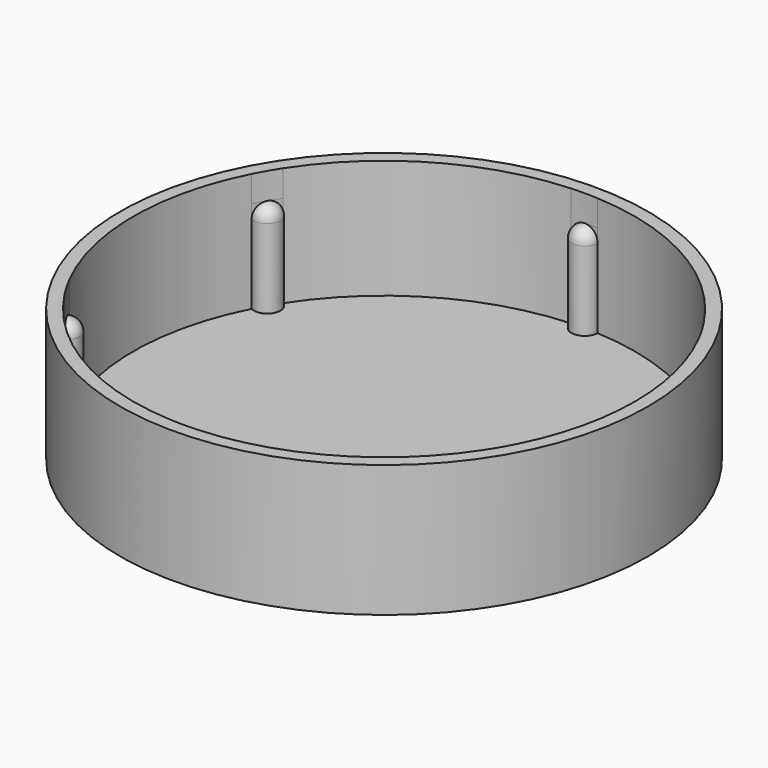
from build123d import *

# Parameters (mm, degrees)
F0_R          = 20
F1_DEPTH      = 9
F2_DEPTH      = 1
F3_DEPTH      = 7
F3_DEPTH_BACK = 1
F4_T4_ANGLE   = 359.64
F4_S5_R       = 19
F4_T6_DEPTH   = 3
F4_T10_ANGLE  = 359.64
F4_S11_R      = 19
F4_T12_DEPTH  = 3
F4_T16_ANGLE  = 359.64
F4_S17_R      = 19
F4_T18_DEPTH  = 3
F4_T22_ANGLE  = 359.64
F4_S23_R      = 19
F4_T24_DEPTH  = 3
F4_T28_ANGLE  = 359.64
F4_S29_R      = 19
F4_T30_DEPTH  = 3
F4_T34_ANGLE  = 359.64
F4_S35_R      = 19
F4_T36_DEPTH  = 3


# Not quite as in the source:
# - a fillet or chamfer that OpenCascade refuses, or shapes differently, is made with other operations: its cross-section is extruded or revolved along the edge and cut away or added


with BuildPart() as f1:
    # F0 (on Top) → F1 (new body)
    with BuildSketch(Plane.XY):
        Circle(F0_R)
        with BuildLine():
            ThreePointArc((16.9315193695, 8.6211166237), (18.4756443463, 4.432895892), (19, 0))
            ThreePointArc((19, 0), (18.4756443463, -4.432895892), (16.9315193695, -8.6211166237))
            ThreePointArc((16.9315193695, -8.6211166237), (16.4544826719, -9.5), (15.9318656899, -10.3525675868))
            ThreePointArc((15.9318656899, -10.3525675868), (9.5, -16.4544826719), (0.9996536796, -18.9736842105))
            ThreePointArc((0.9996536796, -18.9736842105), (0, -19), (-0.9996536796, -18.9736842105))
            ThreePointArc((-0.9996536796, -18.9736842105), (-9.5, -16.4544826719), (-15.9318656899, -10.3525675868))
            ThreePointArc((-15.9318656899, -10.3525675868), (-16.4544826719, -9.5), (-16.9315193695, -8.6211166237))
            ThreePointArc((-16.9315193695, -8.6211166237), (-19, 0), (-16.9315193695, 8.6211166237))
            ThreePointArc((-16.9315193695, 8.6211166237), (-16.4544826719, 9.5), (-15.9318656899, 10.3525675868))
            ThreePointArc((-15.9318656899, 10.3525675868), (-9.5, 16.4544826719), (-0.9996536796, 18.9736842105))
            ThreePointArc((-0.9996536796, 18.9736842105), (0, 19), (0.9996536796, 18.9736842105))
            ThreePointArc((0.9996536796, 18.9736842105), (9.5, 16.4544826719), (15.9318656899, 10.3525675868))
            ThreePointArc((15.9318656899, 10.3525675868), (16.4544826719, 9.5), (16.9315193695, 8.6211166237))
        make_face(mode=Mode.SUBTRACT)
    extrude(amount=F1_DEPTH)

    # F0 (on Top) → F2 (join)
    with BuildSketch(Plane.XY):
        Circle(F0_R)
        with BuildLine():
            ThreePointArc((16.9315193695, 8.6211166237), (18.4756443463, 4.432895892), (19, 0))
            ThreePointArc((19, 0), (18.4756443463, -4.432895892), (16.9315193695, -8.6211166237))
            ThreePointArc((16.9315193695, -8.6211166237), (16.4544826719, -9.5), (15.9318656899, -10.3525675868))
            ThreePointArc((15.9318656899, -10.3525675868), (9.5, -16.4544826719), (0.9996536796, -18.9736842105))
            ThreePointArc((0.9996536796, -18.9736842105), (0, -19), (-0.9996536796, -18.9736842105))
            ThreePointArc((-0.9996536796, -18.9736842105), (-9.5, -16.4544826719), (-15.9318656899, -10.3525675868))
            ThreePointArc((-15.9318656899, -10.3525675868), (-16.4544826719, -9.5), (-16.9315193695, -8.6211166237))
            ThreePointArc((-16.9315193695, -8.6211166237), (-19, 0), (-16.9315193695, 8.6211166237))
            ThreePointArc((-16.9315193695, 8.6211166237), (-16.4544826719, 9.5), (-15.9318656899, 10.3525675868))
            ThreePointArc((-15.9318656899, 10.3525675868), (-9.5, 16.4544826719), (-0.9996536796, 18.9736842105))
            ThreePointArc((-0.9996536796, 18.9736842105), (0, 19), (0.9996536796, 18.9736842105))
            ThreePointArc((0.9996536796, 18.9736842105), (9.5, 16.4544826719), (15.9318656899, 10.3525675868))
            ThreePointArc((15.9318656899, 10.3525675868), (16.4544826719, 9.5), (16.9315193695, 8.6211166237))
        make_face(mode=Mode.SUBTRACT)
        with BuildLine():
            ThreePointArc((16.9315193695, -8.6211166237), (18.4756443463, -4.432895892), (19, 0))
            ThreePointArc((19, 0), (18.4756443463, 4.432895892), (16.9315193695, 8.6211166237))
            ThreePointArc((16.9315193695, 8.6211166237), (15.5884572681, 9), (15.9318656899, 10.3525675868))
            ThreePointArc((15.9318656899, 10.3525675868), (9.5, 16.4544826719), (0.9996536796, 18.9736842105))
            ThreePointArc((0.9996536796, 18.9736842105), (0, 18), (-0.9996536796, 18.9736842105))
            ThreePointArc((-0.9996536796, 18.9736842105), (-9.5, 16.4544826719), (-15.9318656899, 10.3525675868))
            ThreePointArc((-15.9318656899, 10.3525675868), (-15.5884572681, 9), (-16.9315193695, 8.6211166237))
            ThreePointArc((-16.9315193695, 8.6211166237), (-19, 0), (-16.9315193695, -8.6211166237))
            ThreePointArc((-16.9315193695, -8.6211166237), (-15.5884572681, -9), (-15.9318656899, -10.3525675868))
            ThreePointArc((-15.9318656899, -10.3525675868), (-9.5, -16.4544826719), (-0.9996536796, -18.9736842105))
            ThreePointArc((-0.9996536796, -18.9736842105), (0, -18), (0.9996536796, -18.9736842105))
            ThreePointArc((0.9996536796, -18.9736842105), (9.5, -16.4544826719), (15.9318656899, -10.3525675868))
            ThreePointArc((15.9318656899, -10.3525675868), (15.5884572681, -9), (16.9315193695, -8.6211166237))
        make_face()
    extrude(amount=-F2_DEPTH)

    # F0 (on Top) → F3 (join, two sides)
    with BuildSketch(Plane.XY) as f3_sk:
        with BuildLine():
            ThreePointArc((-16.9315193695, 8.6211166237), (-15.5884572681, 9), (-15.9318656899, 10.3525675868))
            ThreePointArc((-15.9318656899, 10.3525675868), (-16.4544826719, 9.5), (-16.9315193695, 8.6211166237))
        make_face()
        with BuildLine():
            ThreePointArc((-0.9996536796, 18.9736842105), (0, 18), (0.9996536796, 18.9736842105))
            ThreePointArc((0.9996536796, 18.9736842105), (0, 19), (-0.9996536796, 18.9736842105))
        make_face()
        with BuildLine():
            ThreePointArc((15.9318656899, 10.3525675868), (15.5884572681, 9), (16.9315193695, 8.6211166237))
            ThreePointArc((16.9315193695, 8.6211166237), (16.4544826719, 9.5), (15.9318656899, 10.3525675868))
        make_face()
        with BuildLine():
            ThreePointArc((15.9318656899, -10.3525675868), (16.4544826719, -9.5), (16.9315193695, -8.6211166237))
            ThreePointArc((16.9315193695, -8.6211166237), (15.5884572681, -9), (15.9318656899, -10.3525675868))
        make_face()
        with BuildLine():
            ThreePointArc((-0.9996536796, -18.9736842105), (0, -19), (0.9996536796, -18.9736842105))
            ThreePointArc((0.9996536796, -18.9736842105), (0, -18), (-0.9996536796, -18.9736842105))
        make_face()
        with BuildLine():
            ThreePointArc((-16.9315193695, -8.6211166237), (-16.4544826719, -9.5), (-15.9318656899, -10.3525675868))
            ThreePointArc((-15.9318656899, -10.3525675868), (-15.5884572681, -9), (-16.9315193695, -8.6211166237))
        make_face()
    extrude(amount=F3_DEPTH)
    extrude(f3_sk.sketch, amount=-F3_DEPTH_BACK)

    # F4: fillet of radius 1 on 6 edges, made by hand


with BuildPart() as f4_tool2:
    # F4_s3 → F4_t4 (revolve)
    with BuildSketch(Plane(origin=(0.0300073325, -0.0515991808, 0), x_dir=(0, 0, 1), z_dir=(0.5027182272, -0.8644503364, 0))):
        with BuildLine():
            ThreePointArc((6, -19.9999062388), (6.7071067812, -19.70701302), (7, -18.9999062388))
            Line((7, -18.9999062388), (7, -19.9999062388))
            Line((7, -19.9999062388), (6, -19.9999062388))
        make_face()
    revolve(axis=Axis((16.4544826719, 9.5, 7), (0, 0, 1)), revolution_arc=F4_T4_ANGLE)

    # F4_s5 → F4_t6 (intersect, symmetric)
    with BuildSketch(Plane.XY.offset(6.5)):
        Circle(F4_S5_R)
    extrude(amount=F4_T6_DEPTH, both=True, mode=Mode.INTERSECT)


with BuildPart() as f1_1:
    add(f1.part)

    # F4_t1: cut F4_tool2
    add(f4_tool2.part, mode=Mode.SUBTRACT)


with BuildPart() as f4_tool8:
    # F4_s9 → F4_t10 (revolve)
    with BuildSketch(Plane(origin=(-0.0296825351, -0.0517867027, 0), x_dir=(0, 0, 1), z_dir=(-0.497276838, -0.8675919239, 0))):
        with BuildLine():
            ThreePointArc((6, -19.9999062388), (6.7071067812, -19.70701302), (7, -18.9999062388))
            Line((7, -18.9999062388), (7, -19.9999062388))
            Line((7, -19.9999062388), (6, -19.9999062388))
        make_face()
    revolve(axis=Axis((16.4544826719, -9.5, 7), (0, 0, 1)), revolution_arc=F4_T10_ANGLE)

    # F4_s11 → F4_t12 (intersect, symmetric)
    with BuildSketch(Plane.XY.offset(6.5)):
        Circle(F4_S11_R)
    extrude(amount=F4_T12_DEPTH, both=True, mode=Mode.INTERSECT)


with BuildPart() as f1_2:
    add(f1_1.part)

    # F4_t7: cut F4_tool8
    add(f4_tool8.part, mode=Mode.SUBTRACT)


with BuildPart() as f4_tool14:
    # F4_s15 → F4_t16 (revolve)
    with BuildSketch(Plane(origin=(-0.0596898677, -0.0001875219, 0), x_dir=(0, 0, 1), z_dir=(-0.9999950652, -0.0031415875, 0))):
        with BuildLine():
            ThreePointArc((6, -19.9999062388), (6.7071067812, -19.70701302), (7, -18.9999062388))
            Line((7, -18.9999062388), (7, -19.9999062388))
            Line((7, -19.9999062388), (6, -19.9999062388))
        make_face()
    revolve(axis=Axis((0, -19, 7), (0, 0, 1)), revolution_arc=F4_T16_ANGLE)

    # F4_s17 → F4_t18 (intersect, symmetric)
    with BuildSketch(Plane.XY.offset(6.5)):
        Circle(F4_S17_R)
    extrude(amount=F4_T18_DEPTH, both=True, mode=Mode.INTERSECT)


with BuildPart() as f1_3:
    add(f1_2.part)

    # F4_t13: cut F4_tool14
    add(f4_tool14.part, mode=Mode.SUBTRACT)


with BuildPart() as f4_tool20:
    # F4_s21 → F4_t22 (revolve)
    with BuildSketch(Plane(origin=(-0.0300073325, 0.0515991808, 0), x_dir=(0, 0, 1), z_dir=(-0.5027182272, 0.8644503364, 0))):
        with BuildLine():
            ThreePointArc((6, -19.9999062388), (6.7071067812, -19.70701302), (7, -18.9999062388))
            Line((7, -18.9999062388), (7, -19.9999062388))
            Line((7, -19.9999062388), (6, -19.9999062388))
        make_face()
    revolve(axis=Axis((-16.4544826719, -9.5, 7), (0, 0, 1)), revolution_arc=F4_T22_ANGLE)

    # F4_s23 → F4_t24 (intersect, symmetric)
    with BuildSketch(Plane.XY.offset(6.5)):
        Circle(F4_S23_R)
    extrude(amount=F4_T24_DEPTH, both=True, mode=Mode.INTERSECT)


with BuildPart() as f1_4:
    add(f1_3.part)

    # F4_t19: cut F4_tool20
    add(f4_tool20.part, mode=Mode.SUBTRACT)


with BuildPart() as f4_tool26:
    # F4_s27 → F4_t28 (revolve)
    with BuildSketch(Plane(origin=(0.0296825351, 0.0517867027, 0), x_dir=(0, 0, 1), z_dir=(0.497276838, 0.8675919239, 0))):
        with BuildLine():
            ThreePointArc((6, -19.9999062388), (6.7071067812, -19.70701302), (7, -18.9999062388))
            Line((7, -18.9999062388), (7, -19.9999062388))
            Line((7, -19.9999062388), (6, -19.9999062388))
        make_face()
    revolve(axis=Axis((-16.4544826719, 9.5, 7), (0, 0, 1)), revolution_arc=F4_T28_ANGLE)

    # F4_s29 → F4_t30 (intersect, symmetric)
    with BuildSketch(Plane.XY.offset(6.5)):
        Circle(F4_S29_R)
    extrude(amount=F4_T30_DEPTH, both=True, mode=Mode.INTERSECT)


with BuildPart() as f1_5:
    add(f1_4.part)

    # F4_t25: cut F4_tool26
    add(f4_tool26.part, mode=Mode.SUBTRACT)


with BuildPart() as f4_tool32:
    # F4_s33 → F4_t34 (revolve)
    with BuildSketch(Plane(origin=(0.0596898677, 0.0001875219, 0), x_dir=(0, 0, 1), z_dir=(0.9999950652, 0.0031415875, 0))):
        with BuildLine():
            ThreePointArc((6, -19.9999062388), (6.7071067812, -19.70701302), (7, -18.9999062388))
            Line((7, -18.9999062388), (7, -19.9999062388))
            Line((7, -19.9999062388), (6, -19.9999062388))
        make_face()
    revolve(axis=Axis((0, 19, 7), (0, 0, 1)), revolution_arc=F4_T34_ANGLE)

    # F4_s35 → F4_t36 (intersect, symmetric)
    with BuildSketch(Plane.XY.offset(6.5)):
        Circle(F4_S35_R)
    extrude(amount=F4_T36_DEPTH, both=True, mode=Mode.INTERSECT)


with BuildPart() as f1_6:
    add(f1_5.part)

    # F4_t31: cut F4_tool32
    add(f4_tool32.part, mode=Mode.SUBTRACT)


solid = f1_6.part
